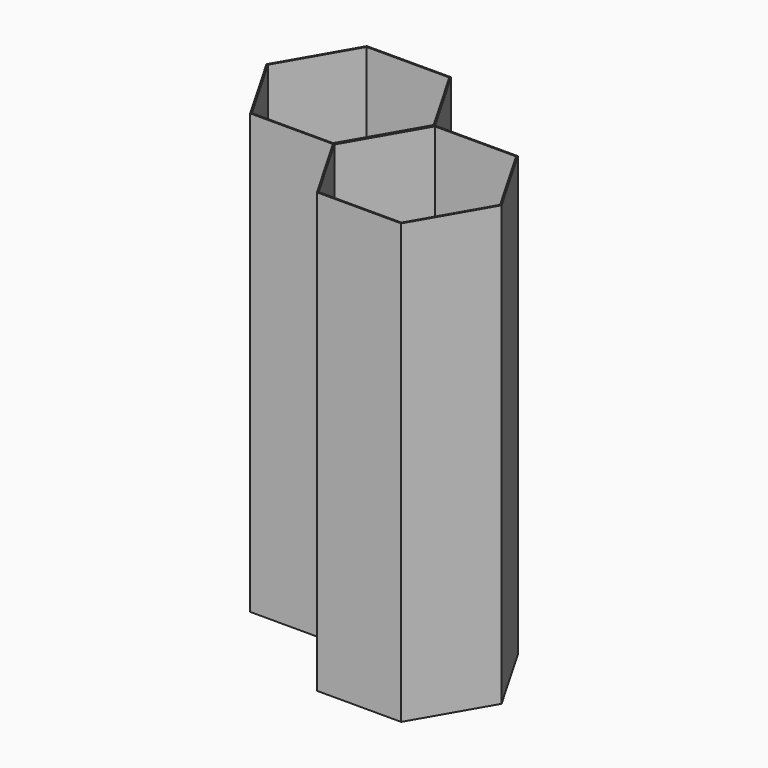
from build123d import *

# Parameters (mm, degrees)
F1_DEPTH = 170
F2_T     = -0.5


# Not quite as in the source:
# - a feature names something its author has since deleted; it is built from what else it names


with BuildPart() as f1:
    # F0 (on Top) → F1 (new body)
    with BuildSketch(Plane.XY):
        Polygon((16.3101451046, 28.25), (-16.3101451046, 28.25), (-32.6202902092, 0), (-16.3101451046, -28.25), (16.3101451046, -28.25), (32.6202902092, 0), align=None)
    extrude(amount=F1_DEPTH)

    # F2
    f2_openings = [f1.faces().sort_by_distance(p)[0] for p in [
        (0, 0, 170),
    ]]
    offset(amount=F2_T, openings=f2_openings)

    # F3: F1 across face


with BuildPart() as f1_1:
    add(f1.part)
    add(f1.part.mirror(Plane(origin=(-24.032204955, 13.875, 85.25), x_dir=(0.5, 0.8660254038, 0), z_dir=(0.8660254038, -0.5, 0))))


solid = f1_1.part
